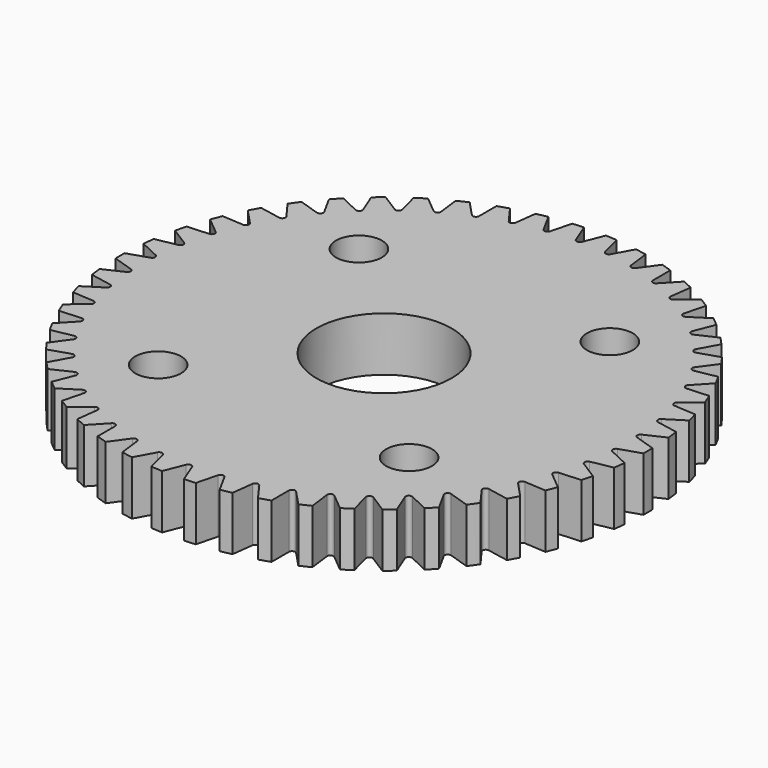
from build123d import *

# Parameters (mm, degrees)
F0_R            = 24.7950019524
F0_R_2          = 2.15265
F0_R_3          = 6.35
F1_DEPTH        = 5.08
F3_DEPTH        = 5.08
F3_COPIES_COUNT = 50


# Not quite as in the source:
# - a pattern or mirror of a feature is missing from the dataset's text; its kind, count and spacing are read off the source's solid
# - a feature names something its author has since deleted; it is built from what else it names


with BuildPart() as f1:
    # F0 (on Top) → F1 (new body)
    with BuildSketch(Plane.XY):
        Circle(F0_R)
        with Locations((-11.7865861589, -11.7865861589)):
            Circle(F0_R_2, mode=Mode.SUBTRACT)
        with Locations((11.7865861589, -11.7865861589)):
            Circle(F0_R_2, mode=Mode.SUBTRACT)
        with Locations((-11.7865861589, 11.7865861589)):
            Circle(F0_R_2, mode=Mode.SUBTRACT)
        Circle(F0_R_3, mode=Mode.SUBTRACT)
        with Locations((11.7865861589, 11.7865861589)):
            Circle(F0_R_2, mode=Mode.SUBTRACT)
    extrude(amount=F1_DEPTH)

    # F2 (on face) → F3 (cut, through all)
    with BuildSketch(Plane.XY.offset(5.08)):
        with BuildLine():
            Line((0.2767116281, 22.8788969552), (1.0256294643, 24.7737806162))
            ThreePointArc((1.0256294643, 24.7737806162), (0, 24.7950019524), (-1.0256294643, 24.7737806162))
            Line((-1.0256294643, 24.7737806162), (-0.2767116281, 22.8788969552))
            ThreePointArc((-0.2767116281, 22.8788969552), (0, 22.6907221018), (0.2767116281, 22.8788969552))
        make_face()
    f3 = extrude(amount=-F3_DEPTH, mode=Mode.SUBTRACT)

    # F3_copies: F3 ×50 about axis
    f3_copies_axis = Axis((0, 0, 0), (0, 0, 1))
    for i in range(1, F3_COPIES_COUNT):
        add(f3.rotate(f3_copies_axis, i * 360 / F3_COPIES_COUNT), mode=Mode.SUBTRACT)


solid = f1.part
